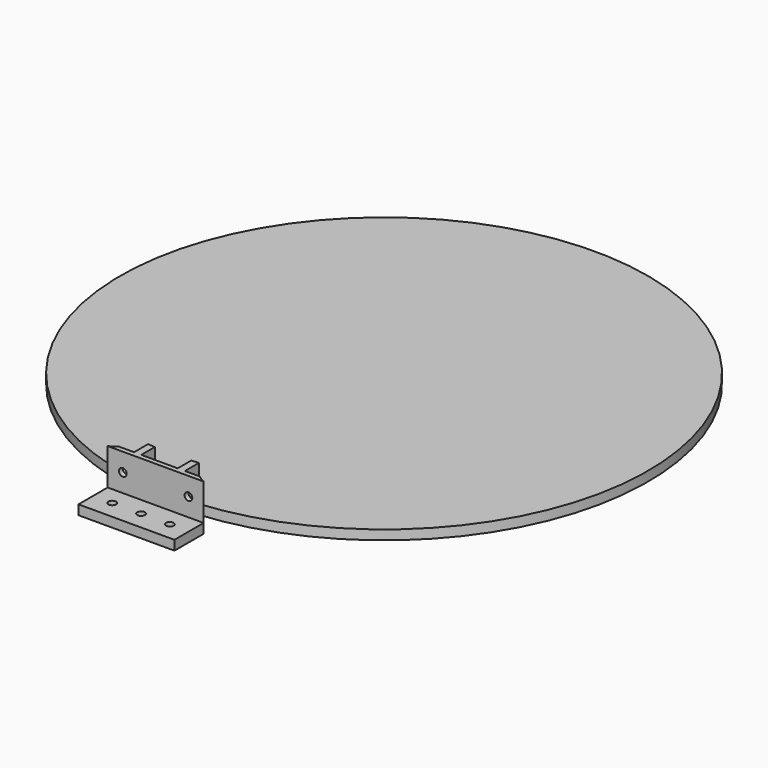
from build123d import *

# Parameters (mm, degrees)
F1_R     = 1.6
F2_DEPTH = 4
F1_W     = 15.2
F1_H     = 2
F3_DEPTH = 19.2
F4_DEPTH = 4
F5_R     = 1.6
F6_DEPTH = 30.601
F7_R     = 1.6
F8_DEPTH = 17.201
F9_DEPTH = 4


# Not quite as in the source:
# - a feature names something its author has since deleted; it is built from what else it names


with BuildPart() as f2:
    # F1 (on Top) → F2 (new body)
    with BuildSketch(Plane.XY):
        Polygon((7.6, -119), (-7.6, -119), (-10.6, -119), (-20, -119), (-20, -134.2), (20, -134.2), (20, -119), (10.6, -119), align=None)
        with Locations((-12, -126.6)):
            Circle(F1_R, mode=Mode.SUBTRACT)
        with Locations((0, -126.6)):
            Circle(F1_R, mode=Mode.SUBTRACT)
        with Locations((12, -126.6)):
            Circle(F1_R, mode=Mode.SUBTRACT)
    extrude(amount=F2_DEPTH)

    # F1 (on Top) → F3 (join)
    with BuildSketch(Plane.XY):
        with BuildLine():
            Line((-7.6, -117), (-7.6, -109.9376186753))
            ThreePointArc((-7.6, -109.9376186753), (-9.1008489139, -109.8235609924), (-10.6, -109.6890149468))
            Line((-10.6, -109.6890149468), (-10.6, -117))
            Line((-10.6, -117), (-10.6, -119))
            Line((-10.6, -119), (-7.6, -119))
            Line((-7.6, -119), (-7.6, -117))
        make_face()
        with BuildLine():
            Line((-10.6, -117), (-16.7608435117, -117))
            ThreePointArc((-16.7608435117, -117), (-18.3217751354, -118.0949827906), (-20, -119))
            Line((-20, -119), (-10.6, -119))
            Line((-10.6, -119), (-10.6, -117))
        make_face()
        with Locations((0, -118)):
            Rectangle(F1_W, F1_H)
        with BuildLine():
            ThreePointArc((10.6, -109.6890149468), (9.1008489139, -109.8235609924), (7.6, -109.9376186753))
            Line((7.6, -109.9376186753), (7.6, -117))
            Line((7.6, -117), (7.6, -119))
            Line((7.6, -119), (10.6, -119))
            Line((10.6, -119), (10.6, -117))
            Line((10.6, -117), (10.6, -109.6890149468))
        make_face()
        with BuildLine():
            ThreePointArc((20, -119), (18.3217751354, -118.0949827906), (16.7608435117, -117))
            Line((16.7608435117, -117), (10.6, -117))
            Line((10.6, -117), (10.6, -119))
            Line((10.6, -119), (20, -119))
        make_face()
    extrude(amount=F3_DEPTH)

    # F1 (on Top) → F4 (join)
    with BuildSketch(Plane.XY):
        with BuildLine():
            ThreePointArc((7.6, -109.9376186753), (0, -110.2), (-7.6, -109.9376186753))
            Line((-7.6, -109.9376186753), (-7.6, -117))
            Line((-7.6, -117), (7.6, -117))
            Line((7.6, -117), (7.6, -109.9376186753))
        make_face()
        with Locations((0, -113.8)):
            Circle(F1_R, mode=Mode.SUBTRACT)
        with BuildLine():
            ThreePointArc((16.7608435117, -117), (13.6040282901, -113.6732968412), (11.5, -109.5983120308))
            ThreePointArc((11.5, -109.5983120308), (11.0500930654, -109.6445869309), (10.6, -109.6890149468))
            Line((10.6, -109.6890149468), (10.6, -117))
            Line((10.6, -117), (16.7608435117, -117))
        make_face()
        with BuildLine():
            ThreePointArc((-10.6, -109.6890149468), (-11.0500930654, -109.6445869309), (-11.5, -109.5983120308))
            ThreePointArc((-11.5, -109.5983120308), (-13.6040282901, -113.6732968412), (-16.7608435117, -117))
            Line((-16.7608435117, -117), (-10.6, -117))
            Line((-10.6, -117), (-10.6, -109.6890149468))
        make_face()
    extrude(amount=F4_DEPTH)

    # F5 (on face) → F6 (cut, through all)
    with BuildSketch(Plane.YZ.offset(10.6)):
        with Locations((-113.3445074734, 11.6)):
            Circle(F5_R)
    extrude(amount=-F6_DEPTH, mode=Mode.SUBTRACT)

    # F7 (on face) → F8 (cut, through all)
    with BuildSketch(Plane(origin=(0, -117, 0), x_dir=(-1, 0, 0), z_dir=(0, 1, 0))):
        with Locations((-13.6804217559, 11.6)):
            Circle(F7_R)
        with Locations((13.6804217559, 11.6)):
            Circle(F7_R)
    extrude(amount=-F8_DEPTH, mode=Mode.SUBTRACT)


with BuildPart() as f9:
    # F1 (on Top) → F9 (new body)
    with BuildSketch(Plane.XY):
        with BuildLine():
            ThreePointArc((9.3920178876, -109.5983120308), (81.0343197899, -74.3870890423), (110, 0))
            ThreePointArc((110, 0), (-74.3870890423, 81.0343197899), (-9.3920178876, -109.5983120308))
            Line((-9.3920178876, -109.5983120308), (-7.6, -109.5983120308))
            Line((-7.6, -109.5983120308), (7.6, -109.5983120308))
            Line((7.6, -109.5983120308), (9.3920178876, -109.5983120308))
        make_face()
        with BuildLine():
            Line((-7.6, -109.5983120308), (-7.6, -109.7371404767))
            ThreePointArc((-7.6, -109.7371404767), (0, -110), (7.6, -109.7371404767))
            Line((7.6, -109.7371404767), (7.6, -109.5983120308))
            Line((7.6, -109.5983120308), (-7.6, -109.5983120308))
        make_face()
        with BuildLine():
            Line((-7.6, -109.5983120308), (-9.3920178876, -109.5983120308))
            ThreePointArc((-9.3920178876, -109.5983120308), (-8.4962925036, -109.6713864857), (-7.6, -109.7371404767))
            Line((-7.6, -109.7371404767), (-7.6, -109.5983120308))
        make_face()
        with BuildLine():
            ThreePointArc((7.6, -109.7371404767), (8.4962925036, -109.6713864857), (9.3920178876, -109.5983120308))
            Line((9.3920178876, -109.5983120308), (7.6, -109.5983120308))
            Line((7.6, -109.5983120308), (7.6, -109.7371404767))
        make_face()
    extrude(amount=F9_DEPTH)


solid = Compound([f2.part, f9.part])
